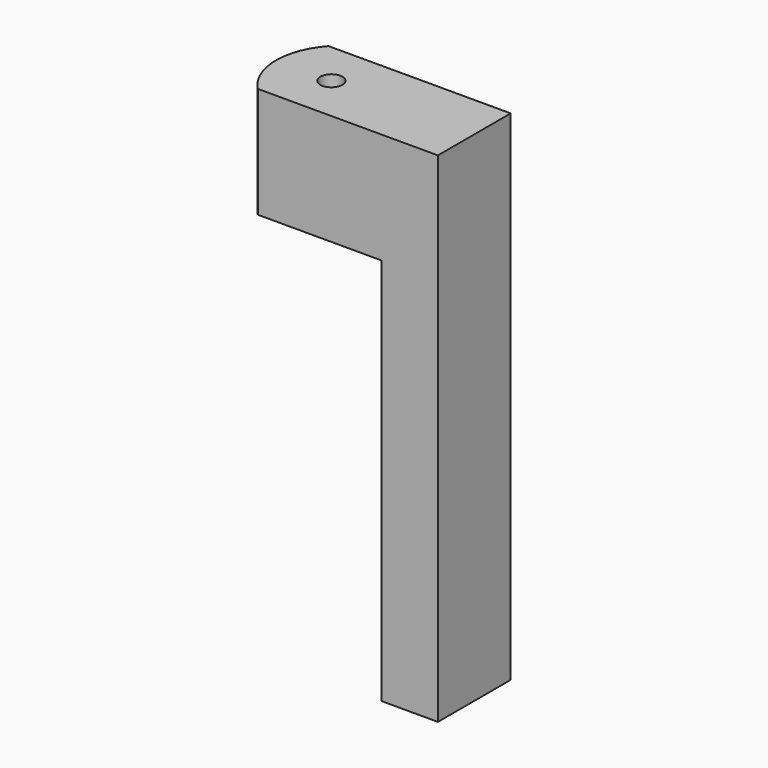
from build123d import *

# Parameters (mm, degrees)
F1_DEPTH = 35
F2_R     = 1
F3_DEPTH = 10


# Not quite as in the source:
# - a feature names something its author has since deleted; it is built from what else it names


with BuildPart() as f1:
    # F0 (on Top) → F1 (new body)
    with BuildSketch(Plane.XY):
        with BuildLine():
            ThreePointArc((-21.369307128, 4.0069422022), (-20.961114092, 2.0219241613), (-20.8242168194, 0))
            ThreePointArc((-20.8242168194, 0), (-20.9750189274, -2.1216319103), (-21.4243930811, -4.2006042786))
            Line((-21.4243930811, -4.2006042786), (-16.3557600736, -4.2006042786))
            Line((-16.3557600736, -4.2006042786), (-16.3557600736, 4.0069422022))
            Line((-16.3557600736, 4.0069422022), (-21.369307128, 4.0069422022))
        make_face()
    extrude(amount=F1_DEPTH)

    # F2 (on face) → F3 (join)
    with BuildSketch(Plane.XY.offset(35)):
        with BuildLine():
            Line((-16.3557600736, -4.2006042786), (-16.3557600736, 4.0069422022))
            Line((-16.3557600736, 4.0069422022), (-21.369307128, 4.0069422022))
            ThreePointArc((-21.369307128, 4.0069422022), (-20.8245546521, -0.1006720692), (-21.4243930811, -4.2006042786))
            Line((-21.4243930811, -4.2006042786), (-16.3557600736, -4.2006042786))
        make_face()
        with BuildLine():
            ThreePointArc((-21.4243930811, -4.2006042786), (-20.8245546521, -0.1006720692), (-21.369307128, 4.0069422022))
            Line((-21.369307128, 4.0069422022), (-32.7901337676, 4.0069422022))
            ThreePointArc((-32.7901337676, 4.0069422022), (-34.3227478364, -0.1327615841), (-32.6084814815, -4.2006042786))
            Line((-32.6084814815, -4.2006042786), (-21.4243930811, -4.2006042786))
        make_face()
        with Locations((-29.3242168194, 0)):
            Circle(F2_R, mode=Mode.SUBTRACT)
    extrude(amount=F3_DEPTH)


solid = f1.part
